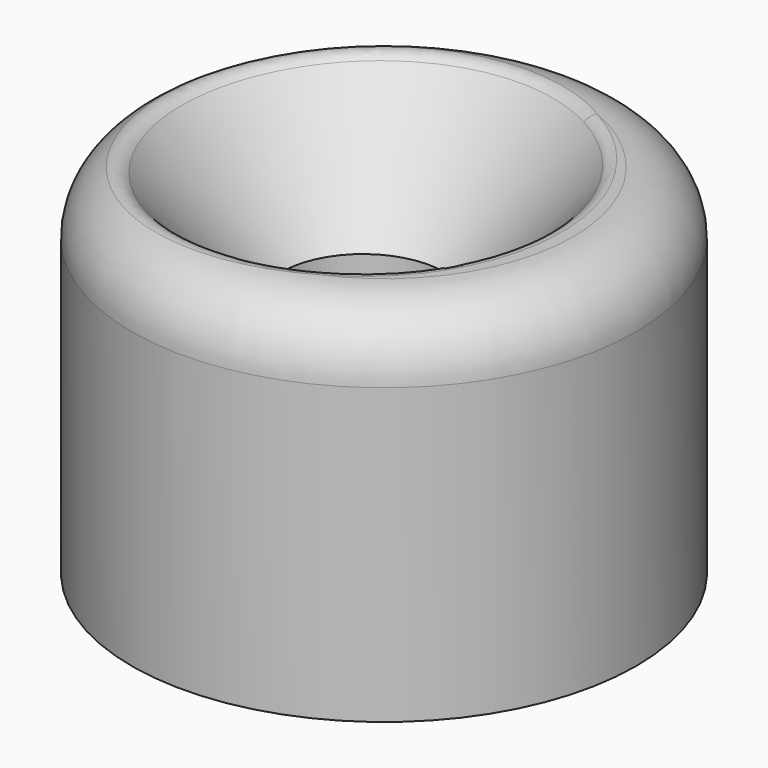
from build123d import *

# Parameters (mm, degrees)
F0_R     = 6
F0_R_2   = 1.95
F1_DEPTH = 8.5
F2_R     = 1.5
F4_R     = 0.35


# Not quite as in the source:
# - a fillet or chamfer that OpenCascade refuses, or shapes differently, is made with other operations: its cross-section is extruded or revolved along the edge and cut away or added


with BuildPart() as f1:
    # F0 (on Top) → F1 (new body)
    with BuildSketch(Plane.XY):
        Circle(F0_R)
        with Locations((-0.5, 0)):
            Circle(F0_R_2, mode=Mode.SUBTRACT)
    extrude(amount=F1_DEPTH)

    # F2
    f2_edges = [f1.edges().sort_by_distance(p)[0] for p in [
        (-6, 0, 8.5),
    ]]
    fillet(f2_edges, radius=F2_R)

    # F3: chamfer of 3 x 2.6078602134 on 1 edges, made by hand

    # F3_s1 → F3_t2 (revolve, cut)
    with BuildSketch(Plane.XZ):
        Polygon((4.0578602134, 8.5), (1.45, 5.5), (1.45, 8.5), align=None)
    revolve(axis=Axis((-0.5, 0, 8.5), (0, 0, 1)), mode=Mode.SUBTRACT)

    # F4
    f4_edges = [f1.edges().sort_by_distance(p)[0] for p in [
        (2.985849, -2.936486, 8.5),
        (2.985849, 2.936486, 8.5),
        (-4.987173, -4e-06, 8.418683),
    ]]
    fillet(f4_edges, radius=F4_R)


solid = f1.part
